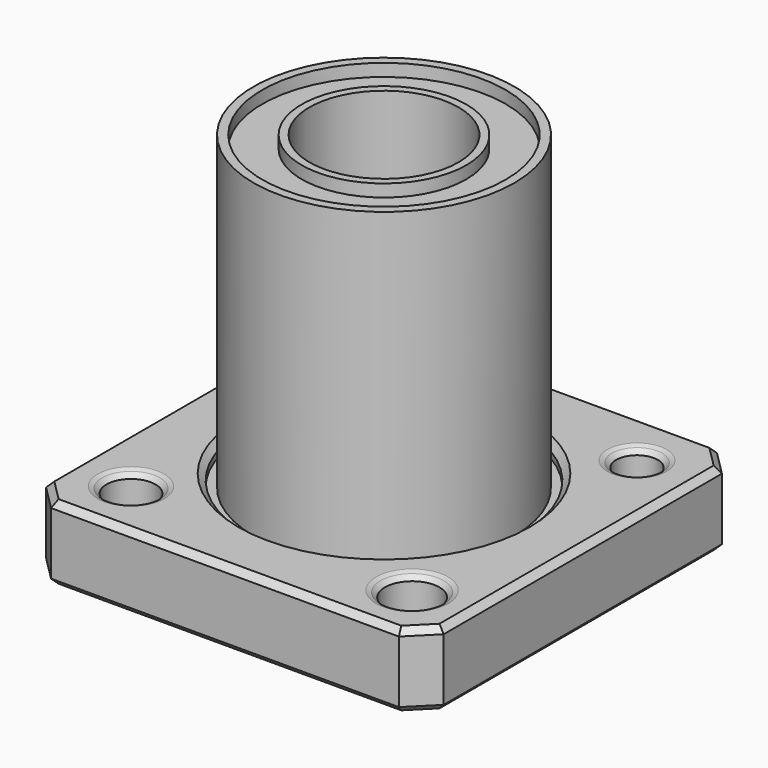
from build123d import *

# Parameters (mm, degrees)
F0_W          = 32
F0_H          = 32
F0_R          = 1.9778790134
F0_R_2        = 2.1975244048
F0_R_3        = 1.8387533056
F0_R_4        = 6
F0_R_5        = 1.6790844608
F1_DEPTH      = 6
F2_R          = 10.5
F2_R_2        = 6
F3_DEPTH      = 24
F4_SIZE       = 2
F5_R          = 11.2136661157
F5_R_2        = 10.5
F6_DEPTH      = 1
F7_R          = 9.7938073019
F7_R_2        = 6.6264369037
F8_DEPTH      = 1
F9_SIZE       = 0.5
F10_R         = 8.3375339565
F10_R_2       = 6.4778965527
F11_DEPTH     = 1
F12_T1_DEPTH  = 30.571682988
F12_T3_DEPTH  = 5.4001101127
F12_T5_DEPTH  = 5.4001101127
F12_T7_DEPTH  = 30.571682988
F12_T9_DEPTH  = 5.4001101127
F12_T11_DEPTH = 5.4001101127


# Not quite as in the source:
# - a fillet or chamfer that OpenCascade refuses, or shapes differently, is made with other operations: its cross-section is extruded or revolved along the edge and cut away or added


with BuildPart() as f1:
    # F0 (on Top) → F1 (new body)
    with BuildSketch(Plane.XY):
        Rectangle(F0_W, F0_H)
        with Locations((-11.313708499, -11.313708499)):
            Circle(F0_R, mode=Mode.SUBTRACT)
        with Locations((11.313708499, -11.313708499)):
            Circle(F0_R_2, mode=Mode.SUBTRACT)
        with Locations((-11.313708499, 11.313708499)):
            Circle(F0_R_3, mode=Mode.SUBTRACT)
        Circle(F0_R_4, mode=Mode.SUBTRACT)
        with Locations((11.313708499, 11.313708499)):
            Circle(F0_R_5, mode=Mode.SUBTRACT)
    extrude(amount=F1_DEPTH)

    # F2 (on face) → F3 (join)
    with BuildSketch(Plane.XY.offset(6)):
        Circle(F2_R)
        Circle(F2_R_2, mode=Mode.SUBTRACT)
    extrude(amount=F3_DEPTH)

    # F4
    f4_edges = [f1.edges().sort_by_distance(p)[0] for p in [
        (-16, -16, 3),
        (16, -16, 3),
        (-16, 16, 3),
        (16, 16, 3),
    ]]
    chamfer(f4_edges, length=F4_SIZE)

    # F5 (on face) → F6 (cut)
    with BuildSketch(Plane.XY.offset(6)):
        Circle(F5_R)
        Circle(F5_R_2, mode=Mode.SUBTRACT)
    extrude(amount=-F6_DEPTH, mode=Mode.SUBTRACT)

    # F7 (on face) → F8 (cut)
    with BuildSketch(Plane.XY.offset(30)):
        Circle(F7_R)
        Circle(F7_R_2, mode=Mode.SUBTRACT)
    extrude(amount=-F8_DEPTH, mode=Mode.SUBTRACT)

    # F9
    f9_edges = [f1.edges().sort_by_distance(p)[0] for p in [
        (-13.291588, -11.313708, 6),
        (9.634624, 11.313708, 6),
        (9.116184, -11.313708, 6),
        (-13.152462, 11.313708, 6),
    ]]
    chamfer(f9_edges, length=F9_SIZE)

    # F10 (on face) → F11 (cut)
    with BuildSketch(Plane(origin=(0, 0, 0), x_dir=(1, 0, 0), z_dir=(0, 0, -1))):
        Circle(F10_R)
        Circle(F10_R_2, mode=Mode.SUBTRACT)
    extrude(amount=-F11_DEPTH, mode=Mode.SUBTRACT)

    # F12: chamfer of 0.5 on 26 edges, made by hand

    # F12_s2 → F12_t1 (cut)
    with BuildSketch(Plane.YZ.offset(-15.285841494)):
        Polygon((-16, 0.5), (-15.5, 0), (-16, 0), align=None)
        Polygon((16, 0.5), (15.5, 0), (16, 0), align=None)
        Polygon((-15.5, 6), (-16, 5.5), (-16, 6), align=None)
        Polygon((15.5, 6), (16, 5.5), (16, 6), align=None)
    extrude(amount=F12_T1_DEPTH, mode=Mode.SUBTRACT)

    # F12_s4 → F12_t3 (cut)
    with BuildSketch(Plane(origin=(1.9092272399, -1.9092272399, 0), x_dir=(0, 0, 1), z_dir=(-0.7071067812, 0.7071067812, 0))):
        Polygon((0.5, -21.2132034356), (0, -20.7132034356), (0, -21.2132034356), align=None)
        Polygon((6, -20.7132034356), (5.5, -21.2132034356), (6, -21.2132034356), align=None)
    extrude(amount=F12_T3_DEPTH, mode=Mode.SUBTRACT)

    # F12_s6 → F12_t5 (cut)
    with BuildSketch(Plane(origin=(-1.9092272399, -1.9092272399, 0), x_dir=(0, 0, 1), z_dir=(0.7071067812, 0.7071067812, 0))):
        Polygon((0.5, 21.2132034356), (0, 20.7132034356), (0, 21.2132034356), align=None)
        Polygon((6, 20.7132034356), (5.5, 21.2132034356), (6, 21.2132034356), align=None)
    extrude(amount=F12_T5_DEPTH, mode=Mode.SUBTRACT)

    # F12_s8 → F12_t7 (cut)
    with BuildSketch(Plane.XZ.offset(-15.285841494)):
        Polygon((-16, 0.5), (-15.5, 0), (-16, 0), align=None)
        Polygon((16, 0.5), (15.5, 0), (16, 0), align=None)
        Polygon((-15.5, 6), (-16, 5.5), (-16, 6), align=None)
        Polygon((15.5, 6), (16, 5.5), (16, 6), align=None)
    extrude(amount=F12_T7_DEPTH, mode=Mode.SUBTRACT)

    # F12_s10 → F12_t9 (cut)
    with BuildSketch(Plane(origin=(1.9092272399, 1.9092272399, 0), x_dir=(0, 0, 1), z_dir=(-0.7071067812, -0.7071067812, 0))):
        Polygon((0.5, 21.2132034356), (0, 20.7132034356), (0, 21.2132034356), align=None)
        Polygon((6, 20.7132034356), (5.5, 21.2132034356), (6, 21.2132034356), align=None)
    extrude(amount=F12_T9_DEPTH, mode=Mode.SUBTRACT)

    # F12_s12 → F12_t11 (cut)
    with BuildSketch(Plane(origin=(-1.9092272399, 1.9092272399, 0), x_dir=(0, 0, 1), z_dir=(0.7071067812, -0.7071067812, 0))):
        Polygon((0.5, -21.2132034356), (0, -20.7132034356), (0, -21.2132034356), align=None)
        Polygon((6, -20.7132034356), (5.5, -21.2132034356), (6, -21.2132034356), align=None)
    extrude(amount=F12_T11_DEPTH, mode=Mode.SUBTRACT)

    # F12_s13 → F12_t14 (revolve, cut)
    with BuildSketch(Plane.XZ.offset(11.313708499)):
        Polygon((-9.3358294856, 0.5), (-8.8358294856, 0), (-9.3358294856, 0), align=None)
    revolve(axis=Axis((-11.313708499, -11.313708499, 0), (0, 0, 1)), mode=Mode.SUBTRACT)

    # F12_s15 → F12_t16 (revolve, cut)
    with BuildSketch(Plane.XZ.offset(11.313708499)):
        Polygon((14.0112329038, 0), (13.5112329038, 0.5), (13.5112329038, 0), align=None)
    revolve(axis=Axis((11.313708499, -11.313708499, 0), (0, 0, 1)), mode=Mode.SUBTRACT)

    # F12_s17 → F12_t18 (revolve, cut)
    with BuildSketch(Plane.XZ):
        Polygon((8.8375339565, 0), (8.3375339565, 0.5), (8.3375339565, 0), align=None)
    revolve(axis=Axis((0, 0, 0), (0, 0, -1)), mode=Mode.SUBTRACT)

    # F12_s19 → F12_t20 (revolve, cut)
    with BuildSketch(Plane.XZ.offset(-11.313708499)):
        Polygon((-8.9749551934, 0), (-9.4749551934, 0.5), (-9.4749551934, 0), align=None)
    revolve(axis=Axis((-11.313708499, 11.313708499, 0), (0, 0, 1)), mode=Mode.SUBTRACT)

    # F12_s21 → F12_t22 (revolve, cut)
    with BuildSketch(Plane.XZ.offset(-11.313708499)):
        Polygon((13.4927929597, 0), (12.9927929597, 0.5), (12.9927929597, 0), align=None)
    revolve(axis=Axis((11.313708499, 11.313708499, 0), (0, 0, 1)), mode=Mode.SUBTRACT)

    # F12_s23 → F12_t24 (revolve, cut)
    with BuildSketch(Plane.XZ.offset(11.313708499)):
        Polygon((-8.6287227044, 6), (-8.982276095, 5.8535533906), (-8.8358294856, 6), align=None)
    revolve(axis=Axis((-11.313708499, -11.313708499, 6), (0, 0, 1)), mode=Mode.SUBTRACT)

    # F12_s25 → F12_t26 (revolve, cut)
    with BuildSketch(Plane.XZ):
        Polygon((11.7136661157, 6), (11.2136661157, 5.5), (11.2136661157, 6), align=None)
    revolve(axis=Axis((0, 0, 6), (0, 0, 1)), mode=Mode.SUBTRACT)

    # F12_s27 → F12_t28 (revolve, cut)
    with BuildSketch(Plane.XZ.offset(-11.313708499)):
        Polygon((13.6998997409, 6), (13.3463463503, 5.8535533906), (13.4927929597, 6), align=None)
    revolve(axis=Axis((11.313708499, 11.313708499, 6), (0, 0, 1)), mode=Mode.SUBTRACT)

    # F12_s29 → F12_t30 (revolve, cut)
    with BuildSketch(Plane.XZ.offset(11.313708499)):
        Polygon((14.218339685, 6), (13.8647862944, 5.8535533906), (14.0112329038, 6), align=None)
    revolve(axis=Axis((11.313708499, -11.313708499, 6), (0, 0, 1)), mode=Mode.SUBTRACT)

    # F12_s31 → F12_t32 (revolve, cut)
    with BuildSketch(Plane.XZ.offset(-11.313708499)):
        Polygon((-8.7678484122, 6), (-9.1214018028, 5.8535533906), (-8.9749551934, 6), align=None)
    revolve(axis=Axis((-11.313708499, 11.313708499, 6), (0, 0, 1)), mode=Mode.SUBTRACT)


solid = f1.part
